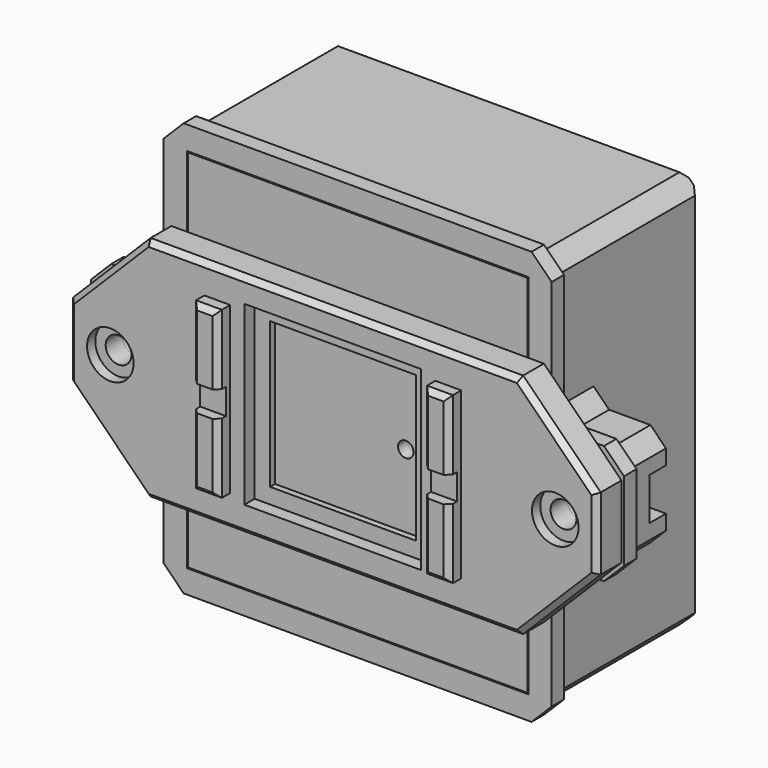
from build123d import *

# Parameters (mm, degrees)
F0_W        = 72
F0_H        = 77
F0_W_2      = 60
F0_H_2      = 65
F1_DEPTH    = 34
F2_W        = 72
F2_H        = 77
F2_W_2      = 51
F2_H_2      = 56
F3_DEPTH    = 3.5
F4_SIZE     = 1
F5_T1_DEPTH = 51.9300979278
F6_W        = 14
F6_H        = 20
F7_DEPTH    = 12
F9_DEPTH    = 4
F10_R       = 2.5
F11_DEPTH   = 37.501
F13_SIZE    = 3
F14_W       = 4
F14_H       = 46.5201788341
F14_W_2     = 63.4782873003
F14_H_2     = 4
F15_DEPTH   = 0.5
F16_R       = 2.5
F16_W       = 60
F16_H       = 65
F17_DEPTH   = 3
F18_W       = 66
F18_H       = 71
F19_DEPTH   = 2
F20_W       = 65.6
F20_H       = 70.6
F21_DEPTH   = 2
F22_W       = 59.4
F22_H       = 64.4
F23_DEPTH   = 1
F24_R       = 1.5
F25_DEPTH   = 37.501
F26_R       = 9.5
F26_R_2     = 7.5
F27_DEPTH   = 1.5
F28_R       = 0.7
F29_W       = 102
F29_H       = 44
F30_DEPTH   = 6
F31_R       = 2.5
F32_DEPTH   = 43.501
F33_R       = 4.5
F34_DEPTH   = 2
F35_SIZE    = 15
F36_W       = 34.2
F36_H       = 34.2
F37_DEPTH   = 2.5
F38_SIZE    = 1
F39_W       = 5
F39_H       = 32
F40_DEPTH   = 3
F41_SIZE    = 1
F42_W       = 96.6998805684
F42_H       = 5
F43_DEPTH   = 2
F44_W       = 28.2
F44_H       = 28.2
F45_DEPTH   = 1.2
F46_R       = 1.5
F47_DEPTH   = 9.001
F48_R       = 9.5
F48_R_2     = 7.5
F49_DEPTH   = 1.2
F50_R       = 0.7


# Not quite as in the source:
# - a fillet or chamfer that OpenCascade refuses, or shapes differently, is made with other operations: its cross-section is extruded or revolved along the edge and cut away or added


with BuildPart() as f1:
    # F0 (on Front) → F1 (new body)
    with BuildSketch(Plane.XZ):
        Rectangle(F0_W, F0_H)
        Rectangle(F0_W_2, F0_H_2, mode=Mode.SUBTRACT)
    extrude(amount=F1_DEPTH)

    # F2 (on face) → F3 (join)
    with BuildSketch(Plane(origin=(0, 0, 0), x_dir=(-1, 0, 0), z_dir=(0, 1, 0))):
        Rectangle(F2_W, F2_H)
        Rectangle(F2_W_2, F2_H_2, mode=Mode.SUBTRACT)
    extrude(amount=F3_DEPTH)

    # F4
    f4_edges = [f1.edges().sort_by_distance(p)[0] for p in [
        (36, 3.5, 0),
        (0, 3.5, -38.5),
        (-36, 3.5, 0),
        (0, 3.5, 38.5),
        (0, 3.5, -28),
        (25.5, 3.5, 0),
        (0, 3.5, 28),
        (-25.5, 3.5, 0),
    ]]
    chamfer(f4_edges, length=F4_SIZE)

    # F5: chamfer of 3 on 4 edges, made by hand

    # F5_s2 → F5_t1 (cut)
    with BuildSketch(Plane.XZ.offset(-10.2150489639)):
        Polygon((-36, 35.5), (-33, 38.5), (-36, 38.5), align=None)
        Polygon((36, 35.5), (33, 38.5), (36, 38.5), align=None)
        Polygon((33, -38.5), (36, -35.5), (36, -38.5), align=None)
        Polygon((-33, -38.5), (-36, -35.5), (-36, -38.5), align=None)
    extrude(amount=F5_T1_DEPTH, mode=Mode.SUBTRACT)

    # F6 (on face) → F7 (join)
    with BuildSketch(Plane.XZ.offset(34)):
        with Locations((-43, 0)):
            Rectangle(F6_W, F6_H)
    extrude(amount=-F7_DEPTH)

    # F8 (on face) → F9 (cut)
    with BuildSketch(Plane(origin=(0, -22, 0), x_dir=(-1, 0, 0), z_dir=(0, 1, 0))):
        Polygon((40.6328638963, -4.1), (45.3671361037, -4.1), (50, -4.1), (50, 4.1), (45.3671361037, 4.1), (40.6328638963, 4.1), (38.2657277926, 0), align=None)
    extrude(amount=-F9_DEPTH, mode=Mode.SUBTRACT)

    # F10 (on face) → F11 (cut, through all)
    with BuildSketch(Plane.XZ.offset(34)):
        with Locations((-43, 0)):
            Circle(F10_R)
    extrude(amount=-F11_DEPTH, mode=Mode.SUBTRACT)

    # F12: F1 across plane


with BuildPart() as f1_1:
    add(f1.part)
    add(f1.part.mirror(Plane.YZ))

    # F13
    f13_edges = [f1_1.edges().sort_by_distance(p)[0] for p in [
        (50, -28, -10),
        (36, -28, -10),
        (50, -28, 10),
        (36, -28, 10),
        (-36, -28, 10),
        (-50, -28, 10),
        (-36, -28, -10),
        (-50, -28, -10),
    ]]
    chamfer(f13_edges, length=F13_SIZE)

    # F14 (on face) → F15 (cut)
    with BuildSketch(Plane(origin=(0, 3.5, 0), x_dir=(-1, 0, 0), z_dir=(0, 1, 0))):
        with Locations((0, 25.2600894171)):
            Rectangle(F14_W, F14_H)
        with Locations((33.7391436501, 0)):
            Rectangle(F14_W_2, F14_H_2)
        Rectangle(F14_W, F14_H_2)
        with Locations((-33.7391436501, 0)):
            Rectangle(F14_W_2, F14_H_2)
        with Locations((0, -25.2600894171)):
            Rectangle(F14_W, F14_H)
    extrude(amount=-F15_DEPTH, mode=Mode.SUBTRACT)

    # F16 (on face) → F17 (join)
    with BuildSketch(Plane.XZ.offset(34)):
        Polygon((-39.6213203436, 11.5), (-47.6213203436, 11.5), (-51.5, 7.6213203436), (-51.5, -7.6213203436), (-47.6213203436, -11.5), (-39.6213203436, -11.5), (-37.5, -13.6213203436), (-37.5, -36.1213203436), (-33.6213203436, -40), (33.6213203436, -40), (37.5, -36.1213203436), (37.5, -13.6213203436), (39.6213203436, -11.5), (47.6213203436, -11.5), (51.5, -7.6213203436), (51.5, 7.6213203436), (47.6213203436, 11.5), (39.6213203436, 11.5), (37.5, 13.6213203436), (37.5, 36.1213203436), (33.6213203436, 40), (-33.6213203436, 40), (-37.5, 36.1213203436), (-37.5, 13.6213203436), align=None)
        with Locations((-43, 0)):
            Circle(F16_R, mode=Mode.SUBTRACT)
        Rectangle(F16_W, F16_H, mode=Mode.SUBTRACT)
        with Locations((43, 0)):
            Circle(F16_R, mode=Mode.SUBTRACT)
    extrude(amount=-F17_DEPTH)

    # F18 (on face) → F19 (cut)
    with BuildSketch(Plane.XZ.offset(34)):
        Rectangle(F18_W, F18_H)
    extrude(amount=-F19_DEPTH, mode=Mode.SUBTRACT)


with BuildPart() as f21:
    # F20 (on face) → F21 (new body, through all)
    with BuildSketch(Plane.XZ.offset(32)):
        Rectangle(F20_W, F20_H)
    extrude(amount=F21_DEPTH)

    # F22 (on face) → F23 (join)
    with BuildSketch(Plane(origin=(0, -32, 0), x_dir=(-1, 0, 0), z_dir=(0, 1, 0))):
        Rectangle(F22_W, F22_H)
    extrude(amount=F23_DEPTH)

    # F24 (on face) → F25 (cut, through all)
    with BuildSketch(Plane.XZ.offset(34)):
        with Locations((11.1516006291, 0)):
            Circle(F24_R)
    extrude(amount=-F25_DEPTH, mode=Mode.SUBTRACT)

    # F26 (on face) → F27 (cut)
    with BuildSketch(Plane.XZ.offset(34)):
        with Locations((11.1516006291, 0)):
            Circle(F26_R)
        with Locations((11.1516006291, 0)):
            Circle(F26_R_2, mode=Mode.SUBTRACT)
    extrude(amount=-F27_DEPTH, mode=Mode.SUBTRACT)

    # F28
    f28_edges = [f21.edges().sort_by_distance(p)[0] for p in [
        (1.651601, -32.5, 0),
        (3.651601, -32.5, 0),
    ]]
    fillet(f28_edges, radius=F28_R)


with BuildPart() as f30:
    # F29 (on face) → F30 (new body)
    with BuildSketch(Plane.XZ.offset(34)):
        with Locations((0, -0.2510596967)):
            Rectangle(F29_W, F29_H)
    extrude(amount=F30_DEPTH)

    # F31 (on face) → F32 (cut, through all)
    with BuildSketch(Plane.XZ.offset(40)):
        with Locations((43, 0)):
            Circle(F31_R)
        with Locations((-43, 0)):
            Circle(F31_R)
    extrude(amount=-F32_DEPTH, mode=Mode.SUBTRACT)

    # F33 (on face) → F34 (cut)
    with BuildSketch(Plane.XZ.offset(40)):
        with Locations((-43, 0)):
            Circle(F33_R)
        with Locations((43, 0)):
            Circle(F33_R)
    extrude(amount=-F34_DEPTH, mode=Mode.SUBTRACT)

    # F35
    f35_edges = [f30.edges().sort_by_distance(p)[0] for p in [
        (-51, -37, -22.25106),
        (51, -37, -22.25106),
        (51, -37, 21.74894),
        (-51, -37, 21.74894),
    ]]
    chamfer(f35_edges, length=F35_SIZE)

    # F36 (on face) → F37 (cut)
    with BuildSketch(Plane.XZ.offset(40)):
        Rectangle(F36_W, F36_H)
    extrude(amount=-F37_DEPTH, mode=Mode.SUBTRACT)

    # F38
    f38_edges = [f30.edges().sort_by_distance(p)[0] for p in [
        (0, -40, -22.25106),
        (-43.5, -40, -14.75106),
        (-51, -40, -0.25106),
        (-43.5, -40, 14.24894),
        (0, -40, 21.74894),
        (43.5, -40, 14.24894),
        (51, -40, -0.25106),
        (43.5, -40, -14.75106),
    ]]
    chamfer(f38_edges, length=F38_SIZE)

    # F39 (on face) → F40 (join)
    with BuildSketch(Plane.XZ.offset(40)):
        with Locations((22.3269723356, 0)):
            Rectangle(F39_W, F39_H)
        with Locations((-22.3269723356, 0)):
            Rectangle(F39_W, F39_H)
    extrude(amount=F40_DEPTH)

    # F41
    f41_edges = [f30.edges().sort_by_distance(p)[0] for p in [
        (19.826972, -43, 0),
        (22.326972, -43, -16),
        (24.826972, -43, 0),
        (22.326972, -43, 16),
        (-22.326972, -43, -16),
        (-19.826972, -43, 0),
        (-22.326972, -43, 16),
        (-24.826972, -43, 0),
    ]]
    chamfer(f41_edges, length=F41_SIZE)

    # F42 (on face) → F43 (cut)
    with BuildSketch(Plane.XZ.offset(43)):
        Rectangle(F42_W, F42_H)
    extrude(amount=-F43_DEPTH, mode=Mode.SUBTRACT)

    # F44 (on face) → F45 (cut)
    with BuildSketch(Plane.XZ.offset(37.5)):
        Rectangle(F44_W, F44_H)
    extrude(amount=-F45_DEPTH, mode=Mode.SUBTRACT)

    # F46 (on face) → F47 (cut, through all)
    with BuildSketch(Plane(origin=(0, -34, 0), x_dir=(-1, 0, 0), z_dir=(0, 1, 0))):
        with Locations((-11.1516006291, 0)):
            Circle(F46_R)
    extrude(amount=-F47_DEPTH, mode=Mode.SUBTRACT)

    # F48 (on face) → F49 (cut)
    with BuildSketch(Plane(origin=(0, -34, 0), x_dir=(-1, 0, 0), z_dir=(0, 1, 0))):
        with Locations((-11.1516006291, 0)):
            Circle(F48_R)
        with Locations((-11.1516006291, 0)):
            Circle(F48_R_2, mode=Mode.SUBTRACT)
    extrude(amount=-F49_DEPTH, mode=Mode.SUBTRACT)

    # F50
    f50_edges = [f30.edges().sort_by_distance(p)[0] for p in [
        (20.651601, -35.2, 0),
        (18.651601, -35.2, 0),
    ]]
    fillet(f50_edges, radius=F50_R)


solid = Compound([f1_1.part, f21.part, f30.part])
